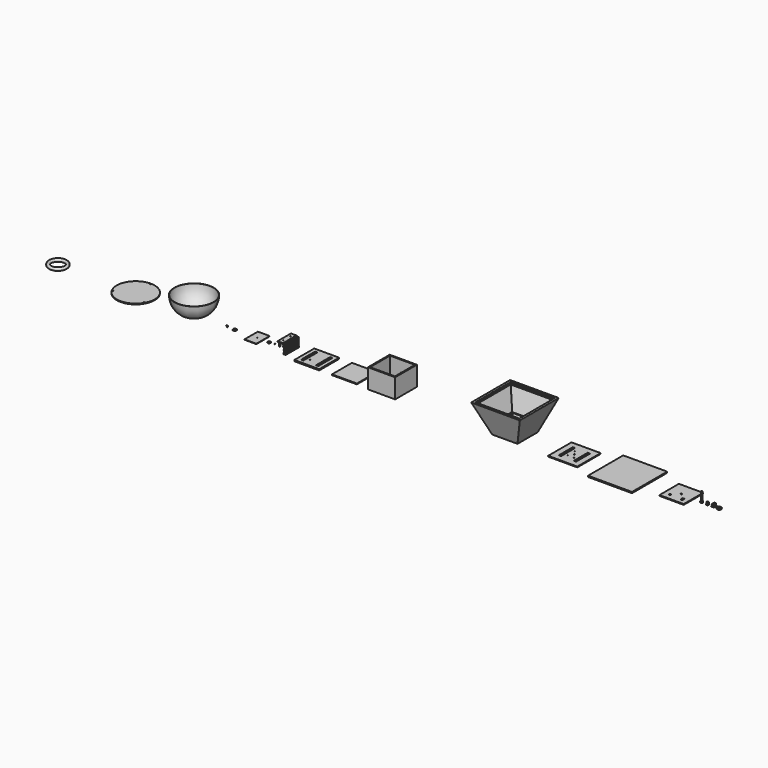
from build123d import *

# Parameters (mm, degrees)
F0_W             = 140
F0_H             = 140
F0_W_2           = 128
F0_H_2           = 128
F1_DEPTH         = 100
F2_W             = 128
F2_H             = 128
F3_DEPTH         = 4
F4_W             = 128
F4_H             = 128
F5_DEPTH         = 6
F6_W             = 12
F6_H             = 90
F7_DEPTH         = 6
F9_DEPTH         = 43
F10_R            = 1.5
F11_DEPTH        = 5
F12_R            = 1.5
F13_DEPTH        = 6
F14_R            = 3
F14_R_2          = 2
F15_DEPTH        = 12
F16_W            = 61
F16_H            = 86
F17_DEPTH        = 2
F19_DEPTH        = 1.5
F20_W            = 5
F20_H            = 7
F21_DEPTH        = 1
F22_R            = 1.5
F23_DEPTH        = 2
F24_R            = 1.5
F25_R            = 1
F26_DEPTH        = 1
F27_R            = 7.5
F28_DEPTH        = 2
F29_R            = 1
F30_DEPTH        = 2
F34_R            = 1
F35_DEPTH        = 3
F36_W            = 20
F36_H            = 2.5
F37_DEPTH        = 3
F37_COPIES_COUNT = 4
F39_W            = 250
F39_H            = 250
F40_DEPTH        = 150
F43_DEPTH        = 250
F44_DEPTH        = 250
F45_W            = 230
F45_H            = 6
F46_DEPTH        = 115
F47_W            = 150
F47_H            = 4
F48_DEPTH        = 75
F51_W            = 125
F51_H            = 4
F52_DEPTH        = 62.5
F49_W            = 226
F49_H            = 226
F50_W            = 106
F50_H            = 106
F55_DEPTH        = 150
F56_W            = 150
F56_H            = 150
F57_DEPTH        = 4
F58_W            = 226
F58_H            = 226
F59_DEPTH        = 6
F60_W            = 12
F60_H            = 90
F61_DEPTH        = 4
F62_R            = 1.5
F62_R_2          = 3
F63_DEPTH        = 4
F64_W            = 125
F64_H            = 125
F65_DEPTH        = 4
F69_R            = 5
F69_W            = 10
F69_H            = 15
F69_R_2          = 3.5
F70_DEPTH        = 4
F74_W            = 14
F74_H            = 19
F75_DEPTH        = 15
F76_W            = 14
F76_H            = 19
F76_W_2          = 10
F76_H_2          = 15
F77_DEPTH        = 10
F78_W            = 14
F78_H            = 19
F78_W_2          = 8
F78_H_2          = 12
F79_DEPTH        = 3
F81_DEPTH        = 8
F85_W            = 4
F85_H            = 1
F86_DEPTH        = 0.5
F90_R            = 97.5
F91_DEPTH        = 4
F92_R            = 2
F93_DEPTH        = 4
F95_DEPTH        = 2.5
F96_R            = 1.5
F97_DEPTH        = 1
F99_R            = 7.5


# Not quite as in the source:
# - a pattern or mirror of a feature is missing from the dataset's text; its kind, count and spacing are read off the source's solid


with BuildPart() as f1:
    # F0 (on Top) → F1 (new body)
    with BuildSketch(Plane.XY):
        with Locations((-280, 0)):
            Rectangle(F0_W, F0_H)
        with Locations((-280, 0)):
            Rectangle(F0_W_2, F0_H_2, mode=Mode.SUBTRACT)
    extrude(amount=F1_DEPTH)

    # F36 (on face) → F37 (cut)
    with BuildSketch(Plane.XZ.offset(-64)):
        with Locations((-280, 41.25)):
            Rectangle(F36_W, F36_H)
    f37 = extrude(amount=-F37_DEPTH, mode=Mode.SUBTRACT)

    # F37_copies: F37 ×4 about axis
    f37_copies_axis = Axis((-280, 0, 0), (0, 0, 1))
    for i in range(1, F37_COPIES_COUNT):
        add(f37.rotate(f37_copies_axis, i * 360 / F37_COPIES_COUNT), mode=Mode.SUBTRACT)


with BuildPart() as f3:
    # F2 (on Top) → F3 (new body)
    with BuildSketch(Plane.XY):
        with Locations((-475.5356311798, 0)):
            Rectangle(F2_W, F2_H)
    extrude(amount=F3_DEPTH)


with BuildPart() as f5:
    # F4 (on Top) → F5 (new body)
    with BuildSketch(Plane.XY):
        with Locations((-669.2357063293, 0)):
            Rectangle(F4_W, F4_H)
    extrude(amount=F5_DEPTH)

    # F6 (on face) → F7 (cut)
    with BuildSketch(Plane.XY.offset(6)):
        with Locations((-707.7357063293, 0)):
            Rectangle(F6_W, F6_H)
        with Locations((-630.7357063293, 0)):
            Rectangle(F6_W, F6_H)
    extrude(amount=-F7_DEPTH, mode=Mode.SUBTRACT)

    # F12 (on face) → F13 (cut)
    with BuildSketch(Plane.XY.offset(6)):
        with Locations((-652.7357063293, 23)):
            Circle(F12_R)
        with Locations((-652.7357063293, -23)):
            Circle(F12_R)
        with Locations((-685.7357063293, 23)):
            Circle(F12_R)
        with Locations((-685.7357063293, -23)):
            Circle(F12_R)
    extrude(amount=-F13_DEPTH, mode=Mode.SUBTRACT)

    # F34 (on face) → F35 (cut)
    with BuildSketch(Plane(origin=(0, 0, 0), x_dir=(1, 0, 0), z_dir=(0, 0, -1))):
        with Locations((-669.2357063293, 58)):
            Circle(F34_R)
        with Locations((-669.2357063293, -58)):
            Circle(F34_R)
        with Locations((-727.2357063293, 0)):
            Circle(F34_R)
        with Locations((-611.2357063293, 0)):
            Circle(F34_R)
    extrude(amount=-F35_DEPTH, mode=Mode.SUBTRACT)


with BuildPart() as f9:
    # F8 (on Front) → F9 (new body, symmetric)
    with BuildSketch(Plane.XZ):
        Polygon((-805.3418579102, 0), (-794.3418579102, 0), (-794.3418579102, 2), (-801.3418579102, 2), (-801.3418579102, 4.5), (-795.3418579102, 4.5), (-795.3418579102, 6), (-801.3418579102, 6), (-801.3418579102, 8.5), (-795.3418579102, 8.5), (-795.3418579102, 10), (-801.3418579102, 10), (-801.3418579102, 12.5), (-795.3418579102, 12.5), (-795.3418579102, 14), (-801.3418579102, 14), (-801.3418579102, 16.5), (-795.3418579102, 16.5), (-795.3418579102, 18), (-801.3418579102, 18), (-801.3418579102, 20.5), (-795.3418579102, 20.5), (-795.3418579102, 22), (-801.3418579102, 22), (-801.3418579102, 24.5), (-795.3418579102, 24.5), (-795.3418579102, 26), (-801.3418579102, 26), (-801.3418579102, 28.5), (-795.3418579102, 28.5), (-795.3418579102, 30), (-801.3418579102, 30), (-801.3418579102, 32.5), (-795.3418579102, 32.5), (-795.3418579102, 34), (-801.3418579102, 34), (-801.3418579102, 36.5), (-795.3418579102, 36.5), (-795.3418579102, 38), (-801.3418579102, 38), (-801.3418579102, 40.5), (-795.3418579102, 40.5), (-795.3418579102, 42), (-801.3418579102, 42), (-801.3418579102, 44.5), (-795.3418579102, 44.5), (-795.3418579102, 46), (-801.3418579102, 46), (-801.3418579102, 50), (-802.3418579102, 50), (-802.3418579102, 49), (-804.3418579102, 49), (-804.3418579102, 50), (-805.3418579102, 50), (-805.3418579102, 49), (-807.3418579102, 49), (-807.3418579102, 50), (-808.3418579102, 50), (-808.3418579102, 49), (-836.3418579102, 49), (-836.3418579102, 44.5), (-803.3418579102, 44.5), (-803.3418579102, 42), (-809.3418579102, 42), (-809.3418579102, 40.5), (-803.3418579102, 40.5), (-803.3418579102, 38), (-809.3418579102, 38), (-809.3418579102, 36.5), (-803.3418579102, 36.5), (-803.3418579102, 34), (-809.3418579102, 34), (-809.3418579102, 32.5), (-803.3418579102, 32.5), (-803.3418579102, 30), (-805.3418579102, 30), (-805.3418579102, 29), (-803.3418579102, 29), (-803.3418579102, 26.5), (-805.3418579102, 26.5), (-805.3418579102, 25.5), (-803.3418579102, 25.5), (-803.3418579102, 23), (-805.3418579102, 23), (-805.3418579102, 22), (-803.3418579102, 22), (-803.3418579102, 19.5), (-805.3418579102, 19.5), (-805.3418579102, 18.5), (-803.3418579102, 18.5), (-803.3418579102, 16), (-805.3418579102, 16), (-805.3418579102, 15), (-803.3418579102, 15), (-803.3418579102, 12.5), (-805.3418579102, 12.5), (-805.3418579102, 11.5), (-803.3418579102, 11.5), (-803.3418579102, 9), (-805.3418579102, 9), (-805.3418579102, 8), (-803.3418579102, 8), (-803.3418579102, 5.5), (-805.3418579102, 5.5), (-805.3418579102, 4.5), (-803.3418579102, 4.5), (-803.3418579102, 2), (-805.3418579102, 2), align=None)
    extrude(amount=F9_DEPTH, both=True)

    # F10 (on face) → F11 (cut)
    with BuildSketch(Plane.XY.offset(49)):
        with Locations((-822.3418579102, 23)):
            Circle(F10_R)
        with Locations((-822.3418579102, -23)):
            Circle(F10_R)
    extrude(amount=-F11_DEPTH, mode=Mode.SUBTRACT)


with BuildPart() as f15:
    # F14 (on Top) → F15 (new body)
    with BuildSketch(Plane.XY):
        with Locations((-860, 0)):
            Circle(F14_R)
        with Locations((-860, 0)):
            Circle(F14_R_2, mode=Mode.SUBTRACT)
    extrude(amount=F15_DEPTH)


with BuildPart() as f17:
    # F16 (on Top) → F17 (new body)
    with BuildSketch(Plane.XY):
        with Locations((-975.7763743401, 0)):
            Rectangle(F16_W, F16_H)
    extrude(amount=F17_DEPTH)

    # F25 (on face) → F26 (cut)
    with BuildSketch(Plane.XY.offset(2)):
        with Locations((-991.6687607765, 32)):
            Circle(F25_R)
        with Locations((-960.9551429749, 32)):
            Circle(F25_R)
        with Locations((-960.9551429749, -32)):
            Circle(F25_R)
        with Locations((-991.6687607765, -32)):
            Circle(F25_R)
        with Locations((-975.7763743401, 0)):
            Circle(F25_R)
    extrude(amount=-F26_DEPTH, mode=Mode.SUBTRACT)


with BuildPart() as f19:
    # F18 (on Top) → F19 (new body)
    with BuildSketch(Plane.XY):
        Polygon((-1079.9999860125, 0), (-1084.9999930063, 8.66025), (-1094.9999930063, 8.66025), (-1100, 0), (-1094.9999930062, -8.66025), (-1084.9999930062, -8.66025), align=None)
    extrude(amount=F19_DEPTH)

    # F20 (on face) → F21 (join)
    with BuildSketch(Plane.XY.offset(1.5)):
        with Locations((-1089.9999930063, 0)):
            Rectangle(F20_W, F20_H)
    extrude(amount=F21_DEPTH)

    # F22 (on face) → F23 (join)
    with BuildSketch(Plane.XY.offset(2.5)):
        with Locations((-1089.9999930063, 0)):
            Circle(F22_R)
    extrude(amount=F23_DEPTH)

    # F24
    f24_edges = [f19.edges().sort_by_distance(p)[0] for p in [
        (-1091.499993, 0, 4.5),
    ]]
    fillet(f24_edges, radius=F24_R)


with BuildPart() as f28:
    # F27 (on Top) → F28 (new body)
    with BuildSketch(Plane.XY):
        with Locations((-914.3823981285, 0)):
            Circle(F27_R)
    extrude(amount=F28_DEPTH)

    # F29 (on face) → F30 (cut)
    with BuildSketch(Plane.XY.offset(2)):
        with Locations((-912.8823981285, 0)):
            Circle(F29_R)
    extrude(amount=-F30_DEPTH, mode=Mode.SUBTRACT)


with BuildPart() as f33:
    # F31 (on Front) → F33 (revolve)
    with BuildSketch(Plane.XZ):
        Polygon((-885, 0), (-884, 0), (-884, 4), (-883, 4), (-883, 5), (-885, 5), align=None)
    revolve(axis=Axis((-885, 0, 2.9777439041), (0, 0, -1)))


with BuildPart() as f40:
    # F39 (on Top) → F40 (new body)
    with BuildSketch(Plane.XY):
        with Locations((350, 0)):
            Rectangle(F39_W, F39_H)
    extrude(amount=F40_DEPTH)

    # F41 (on face) → F43 (cut)
    with BuildSketch(Plane.XZ.offset(125)):
        Polygon((285, 0), (225, 150), (225, 0), align=None)
        Polygon((475, 0), (475, 150), (415, 0), align=None)
    extrude(amount=-F43_DEPTH, mode=Mode.SUBTRACT)

    # F42 (on face) → F44 (cut)
    with BuildSketch(Plane.YZ.offset(475)):
        Polygon((-65, 0), (-125, 150), (-125, 0), align=None)
        Polygon((125, 0), (125, 150), (65, 0), align=None)
    extrude(amount=-F44_DEPTH, mode=Mode.SUBTRACT)

    # F45 (on Front) → F46 (cut, symmetric)
    with BuildSketch(Plane.XZ):
        with Locations((350, 144)):
            Rectangle(F45_W, F45_H)
    extrude(amount=F46_DEPTH, both=True, mode=Mode.SUBTRACT)

    # F47 (on Front) → F48 (cut, symmetric)
    with BuildSketch(Plane.XZ):
        with Locations((350, 44)):
            Rectangle(F47_W, F47_H)
    extrude(amount=F48_DEPTH, both=True, mode=Mode.SUBTRACT)

    # F51 (on Front) → F52 (cut, symmetric)
    with BuildSketch(Plane.XZ):
        with Locations((350, 6)):
            Rectangle(F51_W, F51_H)
    extrude(amount=F52_DEPTH, both=True, mode=Mode.SUBTRACT)

    # F49 (on face) → F53 section 0
    with BuildSketch(Plane.XY.offset(150)):
        with Locations((350, 0)):
            Rectangle(F49_W, F49_H)
    # F50 (on face) → F53 section 1
    with BuildSketch(Plane(origin=(0, 0, 0), x_dir=(1, 0, 0), z_dir=(0, 0, -1))):
        with Locations((350, 0)):
            Rectangle(F50_W, F50_H)
    loft(mode=Mode.SUBTRACT)

    # F54 (on face) → F55 (cut)
    with BuildSketch(Plane.XY.offset(150)):
        Polygon((225.05, 125), (225, 124.95), (349.95, 0), (350, 0.05), align=None)
        Polygon((350, -0.05), (349.95, 0), (225, -124.95), (225.05, -125), align=None)
        Polygon((350, 0.05), (349.95, 0), (350, -0.05), (350.05, 0), align=None)
        Polygon((474.95, 125), (350, 0.05), (350.05, 0), (475, 124.95), align=None)
        Polygon((350.05, 0), (350, -0.05), (474.95, -125), (475, -124.95), align=None)
    extrude(amount=-F55_DEPTH, mode=Mode.SUBTRACT)


with BuildPart() as f57:
    # F56 (on Top) → F57 (new body)
    with BuildSketch(Plane.XY):
        with Locations((655.5882692337, 0)):
            Rectangle(F56_W, F56_H)
    extrude(amount=F57_DEPTH)

    # F60 (on face) → F61 (cut)
    with BuildSketch(Plane.XY.offset(4)):
        with Locations((617.0882692337, 0)):
            Rectangle(F60_W, F60_H)
        with Locations((694.0882692337, 0)):
            Rectangle(F60_W, F60_H)
    extrude(amount=-F61_DEPTH, mode=Mode.SUBTRACT)

    # F62 (on face) → F63 (cut)
    with BuildSketch(Plane.XY.offset(4)):
        with Locations((672.0882692337, 23)):
            Circle(F62_R)
        with Locations((672.0882692337, -23)):
            Circle(F62_R)
        with Locations((639.0882692337, 23)):
            Circle(F62_R)
        with Locations((639.0882692337, -23)):
            Circle(F62_R)
        with Locations((655.5882692337, 0)):
            Circle(F62_R_2)
    extrude(amount=-F63_DEPTH, mode=Mode.SUBTRACT)


with BuildPart() as f59:
    # F58 (on Top) → F59 (new body)
    with BuildSketch(Plane.XY):
        with Locations((929.1037917137, 0)):
            Rectangle(F58_W, F58_H)
    extrude(amount=F59_DEPTH)


with BuildPart() as f65:
    # F64 (on Top) → F65 (new body)
    with BuildSketch(Plane.XY):
        with Locations((1205.2003145218, 0)):
            Rectangle(F64_W, F64_H)
    extrude(amount=F65_DEPTH)

    # F69 (on face) → F70 (cut)
    with BuildSketch(Plane(origin=(0, 0, 0), x_dir=(1, 0, 0), z_dir=(0, 0, -1))):
        with Locations((1172.7003145218, 32.5)):
            Circle(F69_R)
        with Locations((1237.7003145218, 32.5)):
            Rectangle(F69_W, F69_H)
        with Locations((1205.2003145218, 0)):
            Circle(F69_R_2)
    extrude(amount=-F70_DEPTH, mode=Mode.SUBTRACT)


with BuildPart() as f68:
    # F66 (on Front) → F68 (revolve)
    with BuildSketch(Plane.XZ):
        Polygon((1310, 50), (1310, 0), (1316, 0), (1316, 5), (1313, 5), (1313, 50), align=None)
    revolve(axis=Axis((1310, 0, 24.3732246757), (0, 0, -1)))


with BuildPart() as f73:
    # F71 (on Front) → F73 (revolve)
    with BuildSketch(Plane.XZ):
        Polygon((1342.5, 6.5), (1342.5, 0), (1345, 0), (1347, 0), (1347, 2), (1345, 2), (1345, 11), (1340, 11), (1340, 1.5), (1340.5, 1.5), (1340.5, 6.5), align=None)
    revolve(axis=Axis((1340, 0, 5.3871515486), (0, 0, -1)))


with BuildPart() as f75:
    # F74 (on Top) → F75 (new body)
    with BuildSketch(Plane.XY):
        with Locations((1373.2365369797, 0)):
            Rectangle(F74_W, F74_H)
    extrude(amount=F75_DEPTH)

    # F76 (on face) → F77 (cut)
    with BuildSketch(Plane.XY.offset(15)):
        with Locations((1373.2365369797, 0)):
            Rectangle(F76_W, F76_H)
        with Locations((1373.2365369797, 0)):
            Rectangle(F76_W_2, F76_H_2, mode=Mode.SUBTRACT)
    extrude(amount=-F77_DEPTH, mode=Mode.SUBTRACT)

    # F78 (on face) → F79 (cut)
    with BuildSketch(Plane(origin=(0, 0, 0), x_dir=(1, 0, 0), z_dir=(0, 0, -1))):
        with Locations((1373.2365369797, 0)):
            Rectangle(F78_W, F78_H)
        with Locations((1373.2365369797, 0)):
            Rectangle(F78_W_2, F78_H_2, mode=Mode.SUBTRACT)
    extrude(amount=-F79_DEPTH, mode=Mode.SUBTRACT)

    # F80 (on face) → F81 (cut)
    with BuildSketch(Plane.YZ.offset(1377.2365369797)):
        with BuildLine():
            Line((-6, 2.25), (-6, 0))
            Line((-6, 0), (6, 0))
            Line((6, 0), (6, 1))
            ThreePointArc((6, 1), (0.0995289214, 2.5804776455), (-6, 2.25))
        make_face()
    extrude(amount=-F81_DEPTH, mode=Mode.SUBTRACT)


with BuildPart() as f84:
    # F82 (on Front) → F84 (revolve)
    with BuildSketch(Plane.XZ):
        Polygon((1400, 1.5699329088), (1400, 0), (1410, 0), (1411, 4), (1403, 4), (1403, 1.5699329088), align=None)
    revolve(axis=Axis((1400, 0, 1.798098553), (0, 0, -1)))

    # F85 (on face) → F86 (cut)
    with BuildSketch(Plane(origin=(0, 0, 0), x_dir=(1, 0, 0), z_dir=(0, 0, -1))):
        with Locations((1392.0396216966, 0.3893053768)):
            Rectangle(F85_W, F85_H)
    extrude(amount=-F86_DEPTH, mode=Mode.SUBTRACT)


with BuildPart() as f89:
    # F88 (on Front) → F89 (revolve)
    with BuildSketch(Plane.XZ):
        with BuildLine():
            Line((-1300, 0), (-1275, 0))
            ThreePointArc((-1275, 0), (-1220.2306520488, 30.8392172857), (-1199, 90))
            Line((-1199, 90), (-1200, 90))
            ThreePointArc((-1200, 90), (-1220.9358534103, 31.5414495031), (-1275, 1))
            Line((-1275, 1), (-1300, 1))
            Line((-1300, 1), (-1300, 0))
        make_face()
    revolve(axis=Axis((-1300, 0, 74.1855986416), (0, 0, -1)))


with BuildPart() as f91:
    # F90 (on Top) → F91 (new body)
    with BuildSketch(Plane.XY):
        with Locations((-1600, 0)):
            Circle(F90_R)
    extrude(amount=F91_DEPTH)

    # F92 (on face) → F93 (cut)
    with BuildSketch(Plane.XY.offset(4)):
        with Locations((-1600, 92.5)):
            Circle(F92_R)
        with Locations((-1680.1073498501, -46.25)):
            Circle(F92_R)
        with Locations((-1519.8926501499, -46.25)):
            Circle(F92_R)
    extrude(amount=-F93_DEPTH, mode=Mode.SUBTRACT)


with BuildPart() as f95:
    # F94 (on Front) → F95 (new body, symmetric)
    with BuildSketch(Plane.XZ):
        Polygon((-1128.1774463654, 5), (-1128.1774463654, 0), (-1127.1774463654, 0), (-1127.1774463654, 6), (-1134.1774463654, 6), (-1134.1774463654, 5), align=None)
    extrude(amount=F95_DEPTH, both=True)

    # F96 (on face) → F97 (cut)
    with BuildSketch(Plane.XY.offset(6)):
        with Locations((-1131.1774463654, 0)):
            Circle(F96_R)
    extrude(amount=-F97_DEPTH, mode=Mode.SUBTRACT)


with BuildPart() as f100:
    # F99 (on Front) → F100 (revolve)
    with BuildSketch(Plane.XZ):
        with Locations((-1960, 0)):
            Circle(F99_R)
    revolve(axis=Axis((-2000, 0, 37.4013915658), (0, 0, -1)))


solid = Compound([f1.part, f3.part, f5.part, f9.part, f15.part, f17.part, f19.part, f28.part, f33.part, f40.part, f57.part, f59.part, f65.part, f68.part, f73.part, f75.part, f84.part, f89.part, f91.part, f95.part, f100.part])
